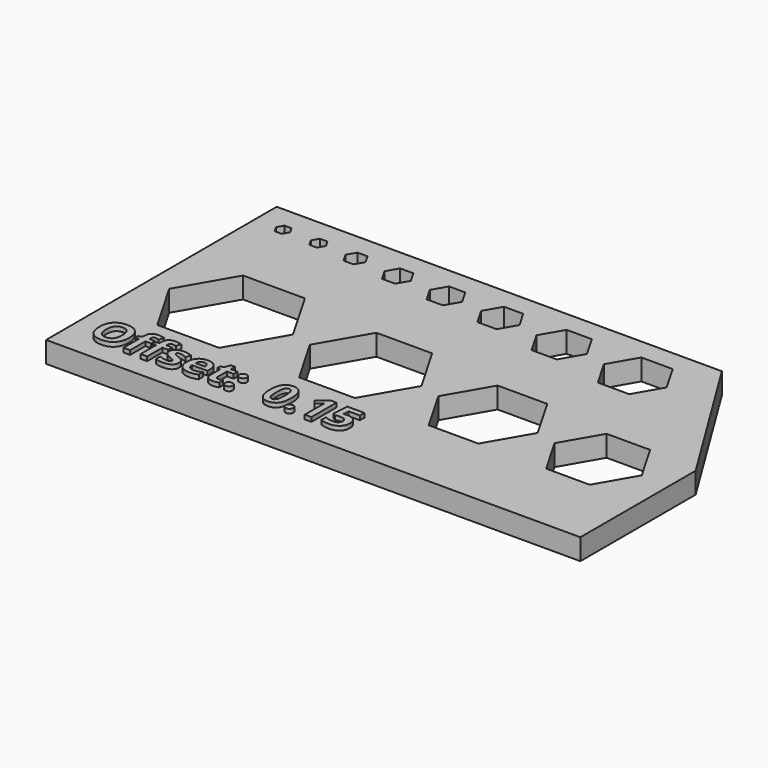
from build123d import *

# Parameters (mm, degrees)
F7_W          = 50.6
F7_H          = 27.3
F8_DEPTH      = 2
F10_TEXT_SIZE = 4.1666666667
F11_DEPTH     = 0.4
F12_SIZE2     = 13.65
F12_SIZE      = 8.4333333333


# Not quite as in the source:
# - Text() gives the source's letters only with a copy of the font that has no kerning and outlines rounded to 1/6400 em; it was checked with that copy


with BuildPart() as f8:
    # F7 (on Top) → F8 (new body)
    with BuildSketch(Plane.XY):
        with Locations((25.3, -13.65)):
            Rectangle(F7_W, F7_H)
        Polygon((10.7901578484, -10.15), (13.7202104645, -15.225), (10.7901578484, -20.3), (4.9300526161, -20.3), (2, -15.225), (4.9300526161, -10.15), align=None, mode=Mode.SUBTRACT)
        Polygon((23.6443429092, -11.15), (26.2857203907, -15.725), (23.6443429092, -20.3), (18.3615879461, -20.3), (15.7202104645, -15.725), (18.3615879461, -11.15), align=None, mode=Mode.SUBTRACT)
        Polygon((35.3438274316, -12.15), (37.6965297785, -16.225), (35.3438274316, -20.3), (30.6384227377, -20.3), (28.2857203907, -16.225), (30.6384227377, -12.15), align=None, mode=Mode.SUBTRACT)
        Polygon((45.8886114156, -13.15), (47.9526386279, -16.725), (45.8886114156, -20.3), (41.7605569909, -20.3), (39.6965297785, -16.725), (41.7605569909, -13.15), align=None, mode=Mode.SUBTRACT)
        Polygon((2.9959292144, -2), (3.3279056191, -2.575), (2.9959292144, -3.15), (2.3319764048, -3.15), (2, -2.575), (2.3319764048, -2), align=None, mode=Mode.SUBTRACT)
        Polygon((6.4104373739, -2), (6.7712812921, -2.625), (6.4104373739, -3.25), (5.6887495374, -3.25), (5.3279056191, -2.625), (5.6887495374, -2), align=None, mode=Mode.SUBTRACT)
        Polygon((10.2002232084, -2), (10.6765371804, -2.825), (10.2002232084, -3.65), (9.2475952642, -3.65), (8.7712812921, -2.825), (9.2475952642, -2), align=None, mode=Mode.SUBTRACT)
        Polygon((24.9470797866, -2), (25.8564064606, -3.575), (24.9470797866, -5.15), (23.1284264386, -5.15), (22.2190997647, -3.575), (23.1284264386, -2), align=None, mode=Mode.SUBTRACT)
        Polygon((14.5384917986, -2), (15.159143338, -3.075), (14.5384917986, -4.15), (13.2971887198, -4.15), (12.6765371804, -3.075), (13.2971887198, -2), align=None, mode=Mode.SUBTRACT)
        Polygon((19.454110658, -2), (20.2190997647, -3.325), (19.454110658, -4.65), (17.9241324446, -4.65), (17.159143338, -3.325), (17.9241324446, -2), align=None, mode=Mode.SUBTRACT)
        Polygon((31.4504118863, -2), (32.6484136948, -4.075), (31.4504118863, -6.15), (29.0544082691, -6.15), (27.8564064606, -4.075), (29.0544082691, -2), align=None, mode=Mode.SUBTRACT)
        Polygon((39.1084445243, -2), (40.5951214675, -4.575), (39.1084445243, -7.15), (36.135090638, -7.15), (34.6484136948, -4.575), (36.135090638, -2), align=None, mode=Mode.SUBTRACT)
    extrude(amount=F8_DEPTH)

    # F10 (on offset) → F11 (join)
    with BuildSketch(Plane.XY.offset(2)):
        with Locations((2, -25.3)):
            Text('Offset:  0.15', F10_TEXT_SIZE, font='Open Sans', font_style=FontStyle.BOLD, text_align=(TextAlign.LEFT, TextAlign.BOTTOM))
    extrude(amount=F11_DEPTH)

    # F12
    f12_edges = [f8.edges().sort_by_distance(p)[0] for p in [
        (50.6, 0, 1),
    ]]
    f12_side = f8.faces().sort_by_distance((25.3, 0, 1))[0]
    chamfer(f12_edges, length=F12_SIZE, length2=F12_SIZE2, reference=f12_side)


solid = f8.part
